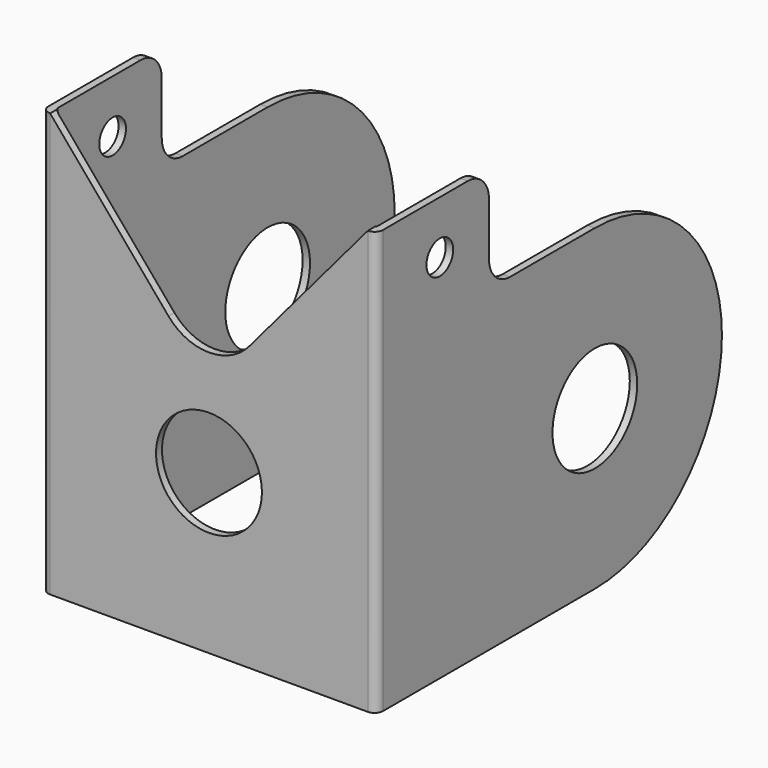
from build123d import *

# Parameters (mm, degrees)
F1_DEPTH = 50.8
F2_R     = 6.35
F3_DEPTH = 25.4
F4_R     = 6.35
F4_R_2   = 2
F5_DEPTH = 40.133


# Not quite as in the source:
# - a feature names something its author has since deleted; it is built from what else it names


with BuildPart() as f1:
    # F0 (on Top) → F1 (new body)
    with BuildSketch(Plane.XY):
        with BuildLine():
            Line((-39.116, 0), (-1.016, 0))
            ThreePointArc((-1.016, 0), (-0.2975795103, 0.2975795103), (0, 1.016))
            Line((0, 1.016), (0, 51.816))
            Line((0, 51.816), (-0.889, 51.816))
            Line((-0.889, 51.816), (-0.889, 1.397))
            ThreePointArc((-0.889, 1.397), (-1.0377897552, 1.0377897552), (-1.397, 0.889))
            Line((-1.397, 0.889), (-38.735, 0.889))
            ThreePointArc((-38.735, 0.889), (-39.0942102448, 1.0377897552), (-39.243, 1.397))
            Line((-39.243, 1.397), (-39.243, 51.816))
            Line((-39.243, 51.816), (-40.132, 51.816))
            Line((-40.132, 51.816), (-40.132, 1.016))
            ThreePointArc((-40.132, 1.016), (-39.8344204897, 0.2975795103), (-39.116, 0))
        make_face()
    extrude(amount=-F1_DEPTH)

    # F2 (on face) → F3 (cut)
    with BuildSketch(Plane.XZ):
        with Locations((-20.066, -31.75)):
            Circle(F2_R)
        with BuildLine():
            Line((-39.116, 0), (-24.915545424, -16.799318136))
            ThreePointArc((-24.915545424, -16.799318136), (-20.066, -19.05), (-15.216454576, -16.799318136))
            Line((-15.216454576, -16.799318136), (-1.016, 0))
            Line((-1.016, 0), (-39.116, 0))
        make_face()
    extrude(amount=-F3_DEPTH, mode=Mode.SUBTRACT)

    # F4 (on face) → F5 (cut, through all)
    with BuildSketch(Plane.YZ):
        with BuildLine():
            ThreePointArc((51.816, -31.75), (46.2363841816, -45.2203841816), (32.766, -50.8))
            Line((32.766, -50.8), (51.816, -50.8))
            Line((51.816, -50.8), (51.816, -31.75))
        make_face()
        with Locations((32.766, -31.75)):
            Circle(F4_R)
        with BuildLine():
            ThreePointArc((32.766, -12.7), (46.2363841816, -18.2796158184), (51.816, -31.75))
            Line((51.816, -31.75), (51.816, 0))
            Line((51.816, 0), (13.716, 0))
            ThreePointArc((13.716, 0), (15.9610640303, -0.9299359697), (16.891, -3.175))
            Line((16.891, -3.175), (16.891, -9.525))
            ThreePointArc((16.891, -9.525), (17.8209359697, -11.7700640303), (20.066, -12.7))
            Line((20.066, -12.7), (32.766, -12.7))
        make_face()
        with Locations((9.525, -6.35)):
            Circle(F4_R_2)
    extrude(amount=-F5_DEPTH, mode=Mode.SUBTRACT)


solid = f1.part
